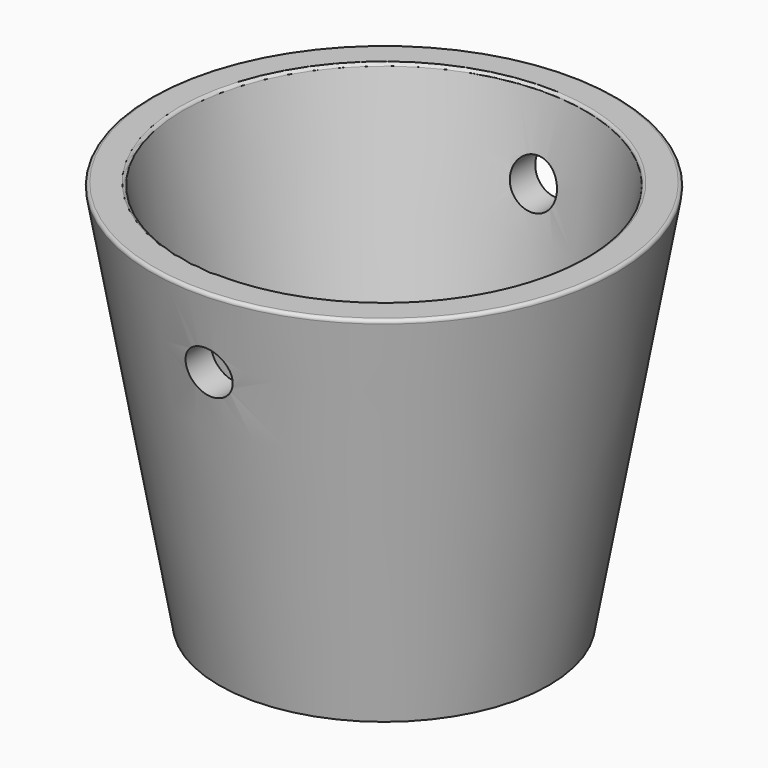
from build123d import *

# Parameters (mm, degrees)
F2_T     = -5.08
F3_R     = 3.81
F4_DEPTH = 51.816
F5_R     = 0.508


with BuildPart() as f1:
    # F0 (on Front) → F1 (revolve)
    with BuildSketch(Plane.XZ):
        Polygon((0, 0), (0, 63.5), (-38.1, 63.5), (-26.903236725, 0), align=None)
    revolve(axis=Axis((0, 0, 31.75), (0, 0, 1)))

    # F2
    f2_openings = [f1.faces().sort_by_distance(p)[0] for p in [
        (0, 0, 63.5),
    ]]
    offset(amount=F2_T, openings=f2_openings)

    # F3 (on Front) → F4 (cut, symmetric)
    with BuildSketch(Plane.XZ):
        with Locations((0, 50.8)):
            Circle(F3_R)
    extrude(amount=F4_DEPTH, both=True, mode=Mode.SUBTRACT)

    # F5
    f5_edges = [f1.edges().sort_by_distance(p)[0] for p in [
        (38.1, 0, 63.5),
        (32.941633, 0, 63.5),
    ]]
    fillet(f5_edges, radius=F5_R)


solid = f1.part
